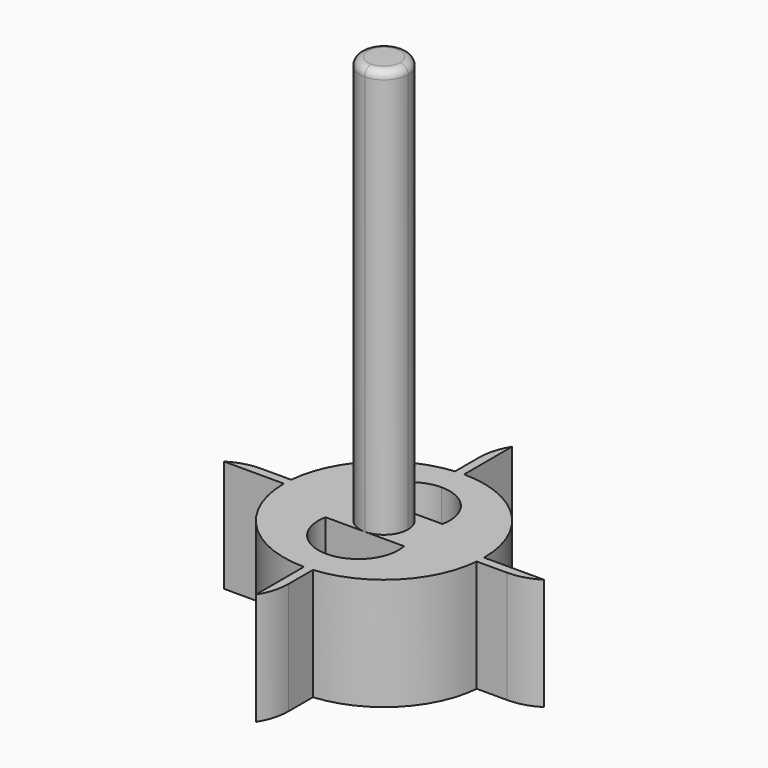
from build123d import *

# Parameters (mm, degrees)
F1_DEPTH = 65
F2_DEPTH = 14
F3_DEPTH = 14
F4_R     = 1
F5_DEPTH = 14


# Not quite as in the source:
# - a feature names something its author has since deleted; it is built from what else it names


with BuildPart() as f1:
    # F0 (on Top) → F1 (new body)
    with BuildSketch(Plane.XY):
        with BuildLine():
            ThreePointArc((0, -3), (2.1213203436, -2.1213203436), (3, 0))
            Line((3, 0), (0, 0))
            Line((0, 0), (0, -3))
        make_face()
        with BuildLine():
            Line((0, 0), (3, 0))
            ThreePointArc((3, 0), (2.1213203436, 2.1213203436), (0, 3))
            Line((0, 3), (0, 0))
        make_face()
        with BuildLine():
            Line((0, 0), (0, 3))
            ThreePointArc((0, 3), (-2.1213203436, 2.1213203436), (-3, 0))
            Line((-3, 0), (0, 0))
        make_face()
        with BuildLine():
            ThreePointArc((-3, 0), (-2.1213203436, -2.1213203436), (0, -3))
            Line((0, -3), (0, 0))
            Line((0, 0), (-3, 0))
        make_face()
    extrude(amount=F1_DEPTH)



with BuildPart() as f2:
    # F0 (on Top) → F2 (new body)
    with BuildSketch(Plane.XY):
        with BuildLine():
            ThreePointArc((-4.8989794856, 3), (-3.8729833462, 7.1622776602), (0, 9))
            Line((0, 9), (0, 12.5))
            ThreePointArc((0, 12.5), (-0.545120999, 12.4881080671), (-1.0892047912, 12.4524548954))
            ThreePointArc((-1.0892047912, 12.4524548954), (-8.8388347648, 8.8388347648), (-12.4524548954, 1.0892047912))
            ThreePointArc((-12.4524548954, 1.0892047912), (-12.4881080671, 0.545120999), (-12.5, 0))
            Line((-12.5, 0), (-4.8989794856, 0))
            Line((-4.8989794856, 0), (-4.8989794856, 3))
        make_face()
        with BuildLine():
            Line((0, -12.5), (0, -9))
            ThreePointArc((0, -9), (-3.8729833462, -7.1622776602), (-4.8989794856, -3))
            Line((-4.8989794856, -3), (-4.8989794856, 0))
            Line((-4.8989794856, 0), (-12.5, 0))
            ThreePointArc((-12.5, 0), (-8.8388347648, -8.8388347648), (0, -12.5))
        make_face()
        with BuildLine():
            Line((12.5, 0), (4.8989794856, 0))
            Line((4.8989794856, 0), (4.8989794856, -3))
            ThreePointArc((4.8989794856, -3), (3.8729833462, -7.1622776602), (0, -9))
            Line((0, -9), (0, -12.5))
            ThreePointArc((0, -12.5), (0.545120999, -12.4881080671), (1.0892047912, -12.4524548954))
            ThreePointArc((1.0892047912, -12.4524548954), (8.8388347648, -8.8388347648), (12.4524548954, -1.0892047912))
            ThreePointArc((12.4524548954, -1.0892047912), (12.4881080671, -0.545120999), (12.5, 0))
        make_face()
        with BuildLine():
            Line((4.8989794856, 3), (4.8989794856, 0))
            Line((4.8989794856, 0), (12.5, 0))
            ThreePointArc((12.5, 0), (8.8388347648, 8.8388347648), (0, 12.5))
            Line((0, 12.5), (0, 9))
            ThreePointArc((0, 9), (3.8729833462, 7.1622776602), (4.8989794856, 3))
        make_face()
    extrude(amount=F2_DEPTH)


with BuildPart() as f1_1:
    add(f1.part)

    add(f2.part)  # F2#2 merges F2
    # F0 (on Top) → F2, piece 2 (join)
    with BuildSketch(Plane.XY):
        with BuildLine():
            ThreePointArc((-3, 0), (-2.1213203436, 2.1213203436), (0, 3))
            Line((0, 3), (-4.8989794856, 3))
            ThreePointArc((-4.8989794856, 3), (-4.2247448714, 1.3257653858), (-3, 0))
        make_face()
        with BuildLine():
            ThreePointArc((0, 3), (2.1213203436, 2.1213203436), (3, 0))
            ThreePointArc((3, 0), (4.2247448714, 1.3257653858), (4.8989794856, 3))
            Line((4.8989794856, 3), (0, 3))
        make_face()
        with BuildLine():
            ThreePointArc((4.8989794856, -3), (4.2247448714, -1.3257653858), (3, 0))
            ThreePointArc((3, 0), (2.1213203436, -2.1213203436), (0, -3))
            Line((0, -3), (4.8989794856, -3))
        make_face()
        with BuildLine():
            Line((-4.8989794856, -3), (0, -3))
            ThreePointArc((0, -3), (-2.1213203436, -2.1213203436), (-3, 0))
            ThreePointArc((-3, 0), (-4.2247448714, -1.3257653858), (-4.8989794856, -3))
        make_face()
    extrude(amount=F2_DEPTH)

    # F0 (on Top) → F3 (join)
    with BuildSketch(Plane.XY):
        with BuildLine():
            Line((20, 0), (12.5, 0))
            ThreePointArc((12.5, 0), (14.2975101103, -0.811390688), (16.25, -1.0892047912))
            ThreePointArc((16.25, -1.0892047912), (18.2024898897, -0.811390688), (20, 0))
        make_face()
        with BuildLine():
            ThreePointArc((-1.0892047912, 16.25), (-0.811390688, 14.2975101103), (0, 12.5))
            Line((0, 12.5), (0, 20))
            ThreePointArc((0, 20), (-0.811390688, 18.2024898897), (-1.0892047912, 16.25))
        make_face()
        with BuildLine():
            Line((-20, 0), (-12.5, 0))
            ThreePointArc((-12.5, 0), (-14.2975101103, 0.811390688), (-16.25, 1.0892047912))
            ThreePointArc((-16.25, 1.0892047912), (-18.2024898897, 0.811390688), (-20, 0))
        make_face()
        with BuildLine():
            ThreePointArc((1.0892047912, -16.25), (0.811390688, -14.2975101103), (0, -12.5))
            Line((0, -12.5), (0, -20))
            ThreePointArc((0, -20), (0.811390688, -18.2024898897), (1.0892047912, -16.25))
        make_face()
        with BuildLine():
            ThreePointArc((16.25, -1.0892047912), (14.2975101103, -0.811390688), (12.5, 0))
            ThreePointArc((12.5, 0), (12.4881080671, -0.545120999), (12.4524548954, -1.0892047912))
            Line((12.4524548954, -1.0892047912), (16.25, -1.0892047912))
        make_face()
        with BuildLine():
            ThreePointArc((-1.0892047912, 12.4524548954), (-0.545120999, 12.4881080671), (0, 12.5))
            ThreePointArc((0, 12.5), (-0.811390688, 14.2975101103), (-1.0892047912, 16.25))
            Line((-1.0892047912, 16.25), (-1.0892047912, 12.4524548954))
        make_face()
        with BuildLine():
            ThreePointArc((-16.25, 1.0892047912), (-14.2975101103, 0.811390688), (-12.5, 0))
            ThreePointArc((-12.5, 0), (-12.4881080671, 0.545120999), (-12.4524548954, 1.0892047912))
            Line((-12.4524548954, 1.0892047912), (-16.25, 1.0892047912))
        make_face()
        with BuildLine():
            ThreePointArc((1.0892047912, -12.4524548954), (0.545120999, -12.4881080671), (0, -12.5))
            ThreePointArc((0, -12.5), (0.811390688, -14.2975101103), (1.0892047912, -16.25))
            Line((1.0892047912, -16.25), (1.0892047912, -12.4524548954))
        make_face()
    extrude(amount=F3_DEPTH)

    # F4
    f4_edges = [f1_1.edges().sort_by_distance(p)[0] for p in [
        (3, 0, 65),
    ]]
    fillet(f4_edges, radius=F4_R)

    # F0 (on Top) → F5 (join)
    with BuildSketch(Plane.XY):
        with BuildLine():
            ThreePointArc((-4.8989794856, -3), (-4.2247448714, -1.3257653858), (-3, 0))
            Line((-3, 0), (-4.8989794856, 0))
            Line((-4.8989794856, 0), (-4.8989794856, -3))
        make_face()
        with BuildLine():
            Line((-4.8989794856, 0), (-3, 0))
            ThreePointArc((-3, 0), (-4.2247448714, 1.3257653858), (-4.8989794856, 3))
            Line((-4.8989794856, 3), (-4.8989794856, 0))
        make_face()
        with BuildLine():
            ThreePointArc((4.8989794856, 3), (4.2247448714, 1.3257653858), (3, 0))
            Line((3, 0), (4.8989794856, 0))
            Line((4.8989794856, 0), (4.8989794856, 3))
        make_face()
        with BuildLine():
            Line((4.8989794856, 0), (3, 0))
            ThreePointArc((3, 0), (4.2247448714, -1.3257653858), (4.8989794856, -3))
            Line((4.8989794856, -3), (4.8989794856, 0))
        make_face()
    extrude(amount=F5_DEPTH)


solid = f1_1.part
